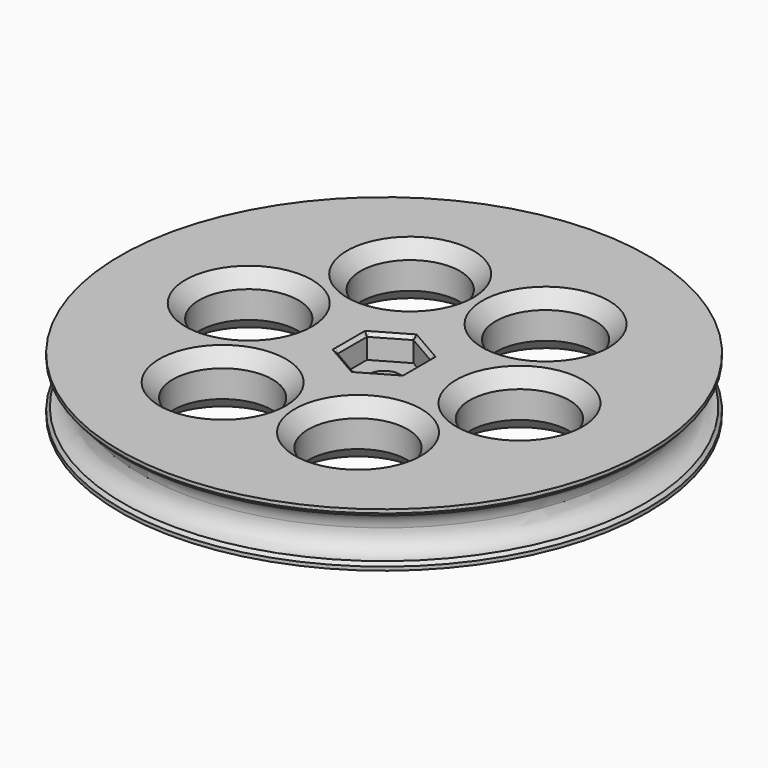
from build123d import *

# Parameters (mm, degrees)
F0_R          = 39
F0_R_2        = 2.325
F1_DEPTH      = 4
F2_R          = 3
F4_R          = 2.325
F5_DEPTH      = 3.5
F6_T4_DEPTH   = 7.9987755183
F6_T10_DEPTH  = 7.9987755183
F6_T16_DEPTH  = 7.9987755183
F6_T22_DEPTH  = 7.9987755183
F6_T28_DEPTH  = 7.9987755183
F6_T34_DEPTH  = 7.9987755183
F6_T38_ANGLE  = 270
F6_T40_ANGLE  = 90
F6_T42_ANGLE  = 90
F6_T44_ANGLE  = 270
F6_T49_DEPTH  = 7.9987755183
F6_T53_DEPTH  = 7.9987755183
F6_T60_DEPTH  = 7.9987755183
F6_T64_DEPTH  = 7.9987755183
F6_T71_DEPTH  = 7.9987755183
F6_T75_DEPTH  = 7.9987755183
F6_T82_DEPTH  = 7.9987755183
F6_T86_DEPTH  = 7.9987755183
F6_T93_DEPTH  = 7.9987755183
F6_T97_DEPTH  = 7.9987755183
F6_T104_DEPTH = 7.9987755183
F6_T108_DEPTH = 7.9987755183
F7_R          = 7.35
F8_DEPTH      = 25
F9_SIZE       = 2


# Not quite as in the source:
# - a fillet or chamfer that OpenCascade refuses, or shapes differently, is made with other operations: its cross-section is extruded or revolved along the edge and cut away or added


with BuildPart() as f1:
    # F0 (on Top) → F1 (new body, symmetric)
    with BuildSketch(Plane.XY):
        Circle(F0_R)
        Circle(F0_R_2, mode=Mode.SUBTRACT)
    extrude(amount=F1_DEPTH, both=True)

    # F2 (on Right) → F3 (revolve, cut)
    with BuildSketch(Plane.YZ):
        with Locations((-39, 0)):
            Circle(F2_R)
    revolve(axis=Axis((0, 0, 0), (0, 0, -1)), mode=Mode.SUBTRACT)

    # F4 (on face) → F5 (cut)
    with BuildSketch(Plane.XY.offset(4)):
        Polygon((-4.7, 2.7135462652), (-4.7, -2.7135462652), (0, -5.4270925304), (4.7, -2.7135462652), (4.7, 2.7135462652), (0, 5.4270925304), align=None)
        Circle(F4_R, mode=Mode.SUBTRACT)
    extrude(amount=-F5_DEPTH, mode=Mode.SUBTRACT)

    # F6: chamfer of 0.5 on 10 edges, made by hand


with BuildPart() as f6_tool2:
    # F6_s3 → F6_t4 (new body)
    with BuildSketch(Plane(origin=(3.463571399, -1.9996938796, 0), x_dir=(0, 0, 1), z_dir=(-0.8660254038, 0.5, 0))):
        Polygon((4, 5.2), (3.5, 4.7), (4, 4.7), align=None)
    extrude(amount=F6_T4_DEPTH)

    split(bisect_by=Plane.YZ.offset(4.7), keep=Keep.BOTTOM)

    split(bisect_by=Plane(origin=(-2.35, 4.0703193978, 0), x_dir=(0, 0, 1), z_dir=(0.5, -0.8660254038, 0)), keep=Keep.TOP)


with BuildPart() as f1_1:
    add(f1.part)

    # F6_t1: cut F6_tool2
    add(f6_tool2.part, mode=Mode.SUBTRACT)


with BuildPart() as f6_tool8:
    # F6_s9 → F6_t10 (new body)
    with BuildSketch(Plane.XZ.offset(3.9993877592)):
        Polygon((5.2, 4), (4.7, 3.5), (4.7, 4), align=None)
    extrude(amount=-F6_T10_DEPTH)

    split(bisect_by=Plane(origin=(2.35, -4.0703193978, 0), x_dir=(0, 0, 1), z_dir=(-0.5, 0.8660254038, 0)), keep=Keep.TOP)

    split(bisect_by=Plane(origin=(2.35, 4.0703193978, 0), x_dir=(0, 0, 1), z_dir=(-0.5, -0.8660254038, 0)), keep=Keep.TOP)


with BuildPart() as f1_2:
    add(f1_1.part)

    # F6_t7: cut F6_tool8
    add(f6_tool8.part, mode=Mode.SUBTRACT)


with BuildPart() as f6_tool14:
    # F6_s15 → F6_t16 (new body)
    with BuildSketch(Plane(origin=(-3.463571399, -1.9996938796, 0), x_dir=(0, 0, 1), z_dir=(0.8660254038, 0.5, 0))):
        Polygon((4, 5.2), (3.5, 4.7), (4, 4.7), align=None)
    extrude(amount=F6_T16_DEPTH)

    split(bisect_by=Plane(origin=(-2.35, -4.0703193978, 0), x_dir=(0, 0, 1), z_dir=(0.5, 0.8660254038, 0)), keep=Keep.TOP)

    split(bisect_by=Plane.YZ.offset(4.7), keep=Keep.BOTTOM)


with BuildPart() as f1_3:
    add(f1_2.part)

    # F6_t13: cut F6_tool14
    add(f6_tool14.part, mode=Mode.SUBTRACT)


with BuildPart() as f6_tool20:
    # F6_s21 → F6_t22 (new body)
    with BuildSketch(Plane(origin=(-3.463571399, 1.9996938796, 0), x_dir=(0, 0, 1), z_dir=(0.8660254038, -0.5, 0))):
        Polygon((4, 5.2), (3.5, 4.7), (4, 4.7), align=None)
    extrude(amount=F6_T22_DEPTH)

    split(bisect_by=Plane.YZ.offset(-4.7), keep=Keep.TOP)

    split(bisect_by=Plane(origin=(2.35, -4.0703193978, 0), x_dir=(0, 0, 1), z_dir=(-0.5, 0.8660254038, 0)), keep=Keep.TOP)


with BuildPart() as f1_4:
    add(f1_3.part)

    # F6_t19: cut F6_tool20
    add(f6_tool20.part, mode=Mode.SUBTRACT)


with BuildPart() as f6_tool26:
    # F6_s27 → F6_t28 (new body)
    with BuildSketch(Plane.XZ.offset(-3.9993877592)):
        Polygon((-5.2, 4), (-4.7, 3.5), (-4.7, 4), align=None)
    extrude(amount=F6_T28_DEPTH)

    split(bisect_by=Plane(origin=(-2.35, -4.0703193978, 0), x_dir=(0, 0, 1), z_dir=(0.5, 0.8660254038, 0)), keep=Keep.TOP)

    split(bisect_by=Plane(origin=(-2.35, 4.0703193978, 0), x_dir=(0, 0, 1), z_dir=(0.5, -0.8660254038, 0)), keep=Keep.TOP)


with BuildPart() as f1_5:
    add(f1_4.part)

    # F6_t25: cut F6_tool26
    add(f6_tool26.part, mode=Mode.SUBTRACT)


with BuildPart() as f6_tool32:
    # F6_s33 → F6_t34 (new body)
    with BuildSketch(Plane(origin=(3.463571399, 1.9996938796, 0), x_dir=(0, 0, 1), z_dir=(-0.8660254038, -0.5, 0))):
        Polygon((4, 5.2), (3.5, 4.7), (4, 4.7), align=None)
    extrude(amount=F6_T34_DEPTH)

    split(bisect_by=Plane.YZ.offset(-4.7), keep=Keep.TOP)

    split(bisect_by=Plane(origin=(2.35, 4.0703193978, 0), x_dir=(0, 0, 1), z_dir=(-0.5, -0.8660254038, 0)), keep=Keep.TOP)


with BuildPart() as f1_6:
    add(f1_5.part)

    # F6_t31: cut F6_tool32
    add(f6_tool32.part, mode=Mode.SUBTRACT)

    # F6_s37 → F6_t38 (revolve, cut)
    with BuildSketch(Plane.YZ):
        with BuildLine():
            Line((-39, -3.4641016151), (-38.5714285714, -2.9692299558))
            ThreePointArc((-38.5714285714, -2.9692299558), (-38.7780755038, -2.9917803258), (-39, -3))
            Line((-39, -3), (-39, -3.4641016151))
        make_face()
    revolve(axis=Axis((0, 0, -3), (0, 0, -1)), revolution_arc=F6_T38_ANGLE, mode=Mode.SUBTRACT)

    # F6_s39 → F6_t40 (revolve, cut)
    with BuildSketch(Plane.XZ):
        with BuildLine():
            Line((39, -3.4641016151), (38.5714285714, -2.9692299558))
            ThreePointArc((38.5714285714, -2.9692299558), (38.7780755038, -2.9917803258), (39, -3))
            Line((39, -3), (39, -3.4641016151))
        make_face()
    revolve(axis=Axis((0, 0, -3), (0, 0, -1)), revolution_arc=F6_T40_ANGLE, mode=Mode.SUBTRACT)

    # F6_s41 → F6_t42 (revolve, cut)
    with BuildSketch(Plane.XZ):
        with BuildLine():
            Line((38.5714285714, 2.9692299558), (39, 3.4641016151))
            Line((39, 3.4641016151), (39, 3))
            ThreePointArc((39, 3), (38.7780755038, 2.9917803258), (38.5714285714, 2.9692299558))
        make_face()
    revolve(axis=Axis((0, 0, 3), (0, 0, -1)), revolution_arc=F6_T42_ANGLE, mode=Mode.SUBTRACT)

    # F6_s43 → F6_t44 (revolve, cut)
    with BuildSketch(Plane.YZ):
        with BuildLine():
            Line((-38.5714285714, 2.9692299558), (-39, 3.4641016151))
            Line((-39, 3.4641016151), (-39, 3))
            ThreePointArc((-39, 3), (-38.7780755038, 2.9917803258), (-38.5714285714, 2.9692299558))
        make_face()
    revolve(axis=Axis((0, 0, 3), (0, 0, -1)), revolution_arc=F6_T44_ANGLE, mode=Mode.SUBTRACT)


with BuildPart() as f6_tool47:
    # F6_s48 → F6_t49 (new body)
    with BuildSketch(Plane.XZ.offset(3.9993877592)):
        Polygon((5.2, 4), (4.7, 3.5), (4.7, 4), align=None)
    extrude(amount=-F6_T49_DEPTH)

    split(bisect_by=Plane(origin=(2.35, 4.0703193978, 0), x_dir=(0, 0, 1), z_dir=(0.5, 0.8660254038, 0)), keep=Keep.TOP)


with BuildPart() as f6_tool51:
    # F6_s52 → F6_t53 (new body)
    with BuildSketch(Plane(origin=(3.463571399, -1.9996938796, 0), x_dir=(0, 0, 1), z_dir=(-0.8660254038, 0.5, 0))):
        Polygon((4, 5.2), (3.5, 4.7), (4, 4.7), align=None)
    extrude(amount=F6_T53_DEPTH)

    split(bisect_by=Plane.YZ.offset(4.7), keep=Keep.TOP)


with BuildPart() as f6_tool47_1:
    add(f6_tool47.part)

    # F6_t55: intersect F6_tool51
    add(f6_tool51.part, mode=Mode.INTERSECT)


with BuildPart() as f1_7:
    add(f1_6.part)

    # F6_t45: cut F6_tool47
    add(f6_tool47_1.part, mode=Mode.SUBTRACT)


with BuildPart() as f6_tool58:
    # F6_s59 → F6_t60 (new body)
    with BuildSketch(Plane(origin=(3.463571399, -1.9996938796, 0), x_dir=(0, 0, 1), z_dir=(-0.8660254038, 0.5, 0))):
        Polygon((4, 5.2), (3.5, 4.7), (4, 4.7), align=None)
    extrude(amount=F6_T60_DEPTH)

    split(bisect_by=Plane(origin=(-2.35, 4.0703193978, 0), x_dir=(0, 0, 1), z_dir=(-0.5, 0.8660254038, 0)), keep=Keep.TOP)


with BuildPart() as f6_tool62:
    # F6_s63 → F6_t64 (new body)
    with BuildSketch(Plane(origin=(3.463571399, 1.9996938796, 0), x_dir=(0, 0, 1), z_dir=(-0.8660254038, -0.5, 0))):
        Polygon((4, 5.2), (3.5, 4.7), (4, 4.7), align=None)
    extrude(amount=F6_T64_DEPTH)

    split(bisect_by=Plane(origin=(2.35, 4.0703193978, 0), x_dir=(0, 0, 1), z_dir=(0.5, 0.8660254038, 0)), keep=Keep.TOP)


with BuildPart() as f6_tool58_1:
    add(f6_tool58.part)

    # F6_t66: intersect F6_tool62
    add(f6_tool62.part, mode=Mode.INTERSECT)


with BuildPart() as f1_8:
    add(f1_7.part)

    # F6_t56: cut F6_tool58
    add(f6_tool58_1.part, mode=Mode.SUBTRACT)


with BuildPart() as f6_tool69:
    # F6_s70 → F6_t71 (new body)
    with BuildSketch(Plane(origin=(-3.463571399, -1.9996938796, 0), x_dir=(0, 0, 1), z_dir=(0.8660254038, 0.5, 0))):
        Polygon((4, 5.2), (3.5, 4.7), (4, 4.7), align=None)
    extrude(amount=F6_T71_DEPTH)

    split(bisect_by=Plane.YZ.offset(4.7), keep=Keep.TOP)


with BuildPart() as f6_tool73:
    # F6_s74 → F6_t75 (new body)
    with BuildSketch(Plane.XZ.offset(3.9993877592)):
        Polygon((5.2, 4), (4.7, 3.5), (4.7, 4), align=None)
    extrude(amount=-F6_T75_DEPTH)

    split(bisect_by=Plane(origin=(2.35, -4.0703193978, 0), x_dir=(0, 0, 1), z_dir=(0.5, -0.8660254038, 0)), keep=Keep.TOP)


with BuildPart() as f6_tool69_1:
    add(f6_tool69.part)

    # F6_t77: intersect F6_tool73
    add(f6_tool73.part, mode=Mode.INTERSECT)


with BuildPart() as f1_9:
    add(f1_8.part)

    # F6_t67: cut F6_tool69
    add(f6_tool69_1.part, mode=Mode.SUBTRACT)


with BuildPart() as f6_tool80:
    # F6_s81 → F6_t82 (new body)
    with BuildSketch(Plane(origin=(-3.463571399, 1.9996938796, 0), x_dir=(0, 0, 1), z_dir=(0.8660254038, -0.5, 0))):
        Polygon((4, 5.2), (3.5, 4.7), (4, 4.7), align=None)
    extrude(amount=F6_T82_DEPTH)

    split(bisect_by=Plane(origin=(2.35, -4.0703193978, 0), x_dir=(0, 0, 1), z_dir=(0.5, -0.8660254038, 0)), keep=Keep.TOP)


with BuildPart() as f6_tool84:
    # F6_s85 → F6_t86 (new body)
    with BuildSketch(Plane(origin=(-3.463571399, -1.9996938796, 0), x_dir=(0, 0, 1), z_dir=(0.8660254038, 0.5, 0))):
        Polygon((4, 5.2), (3.5, 4.7), (4, 4.7), align=None)
    extrude(amount=F6_T86_DEPTH)

    split(bisect_by=Plane(origin=(-2.35, -4.0703193978, 0), x_dir=(0, 0, 1), z_dir=(-0.5, -0.8660254038, 0)), keep=Keep.TOP)


with BuildPart() as f6_tool80_1:
    add(f6_tool80.part)

    # F6_t88: intersect F6_tool84
    add(f6_tool84.part, mode=Mode.INTERSECT)


with BuildPart() as f1_10:
    add(f1_9.part)

    # F6_t78: cut F6_tool80
    add(f6_tool80_1.part, mode=Mode.SUBTRACT)


with BuildPart() as f6_tool91:
    # F6_s92 → F6_t93 (new body)
    with BuildSketch(Plane.XZ.offset(-3.9993877592)):
        Polygon((-5.2, 4), (-4.7, 3.5), (-4.7, 4), align=None)
    extrude(amount=F6_T93_DEPTH)

    split(bisect_by=Plane(origin=(-2.35, -4.0703193978, 0), x_dir=(0, 0, 1), z_dir=(-0.5, -0.8660254038, 0)), keep=Keep.TOP)


with BuildPart() as f6_tool95:
    # F6_s96 → F6_t97 (new body)
    with BuildSketch(Plane(origin=(-3.463571399, 1.9996938796, 0), x_dir=(0, 0, 1), z_dir=(0.8660254038, -0.5, 0))):
        Polygon((4, 5.2), (3.5, 4.7), (4, 4.7), align=None)
    extrude(amount=F6_T97_DEPTH)

    split(bisect_by=Plane.YZ.offset(-4.7), keep=Keep.BOTTOM)


with BuildPart() as f6_tool91_1:
    add(f6_tool91.part)

    # F6_t99: intersect F6_tool95
    add(f6_tool95.part, mode=Mode.INTERSECT)


with BuildPart() as f1_11:
    add(f1_10.part)

    # F6_t89: cut F6_tool91
    add(f6_tool91_1.part, mode=Mode.SUBTRACT)


with BuildPart() as f6_tool102:
    # F6_s103 → F6_t104 (new body)
    with BuildSketch(Plane.XZ.offset(-3.9993877592)):
        Polygon((-5.2, 4), (-4.7, 3.5), (-4.7, 4), align=None)
    extrude(amount=F6_T104_DEPTH)

    split(bisect_by=Plane(origin=(-2.35, 4.0703193978, 0), x_dir=(0, 0, 1), z_dir=(-0.5, 0.8660254038, 0)), keep=Keep.TOP)


with BuildPart() as f6_tool106:
    # F6_s107 → F6_t108 (new body)
    with BuildSketch(Plane(origin=(3.463571399, 1.9996938796, 0), x_dir=(0, 0, 1), z_dir=(-0.8660254038, -0.5, 0))):
        Polygon((4, 5.2), (3.5, 4.7), (4, 4.7), align=None)
    extrude(amount=F6_T108_DEPTH)

    split(bisect_by=Plane.YZ.offset(-4.7), keep=Keep.BOTTOM)


with BuildPart() as f6_tool102_1:
    add(f6_tool102.part)

    # F6_t110: intersect F6_tool106
    add(f6_tool106.part, mode=Mode.INTERSECT)


with BuildPart() as f1_12:
    add(f1_11.part)

    # F6_t100: cut F6_tool102
    add(f6_tool102_1.part, mode=Mode.SUBTRACT)

    # F7 (on face) → F8 (cut)
    with BuildSketch(Plane.XY.offset(4)):
        with Locations((20, 0)):
            Circle(F7_R)
        with Locations((10, -17.3205080757)):
            Circle(F7_R)
        with Locations((-10, -17.3205080757)):
            Circle(F7_R)
        with Locations((-20, 0)):
            Circle(F7_R)
        with Locations((-10, 17.3205080757)):
            Circle(F7_R)
        with Locations((10, 17.3205080757)):
            Circle(F7_R)
    extrude(amount=-F8_DEPTH, mode=Mode.SUBTRACT)

    # F9
    f9_edges = [f1_12.edges().sort_by_distance(p)[0] for p in [
        (12.65, 0, 4),
        (2.65, -17.320508, 4),
        (-17.35, -17.320508, 4),
        (-27.35, 0, 4),
        (-17.35, 17.320508, 4),
        (2.65, 17.320508, 4),
        (-27.35, 0, -4),
        (-17.35, -17.320508, -4),
        (2.65, -17.320508, -4),
        (12.65, 0, -4),
        (2.65, 17.320508, -4),
        (-17.35, 17.320508, -4),
    ]]
    chamfer(f9_edges, length=F9_SIZE)


solid = f1_12.part
